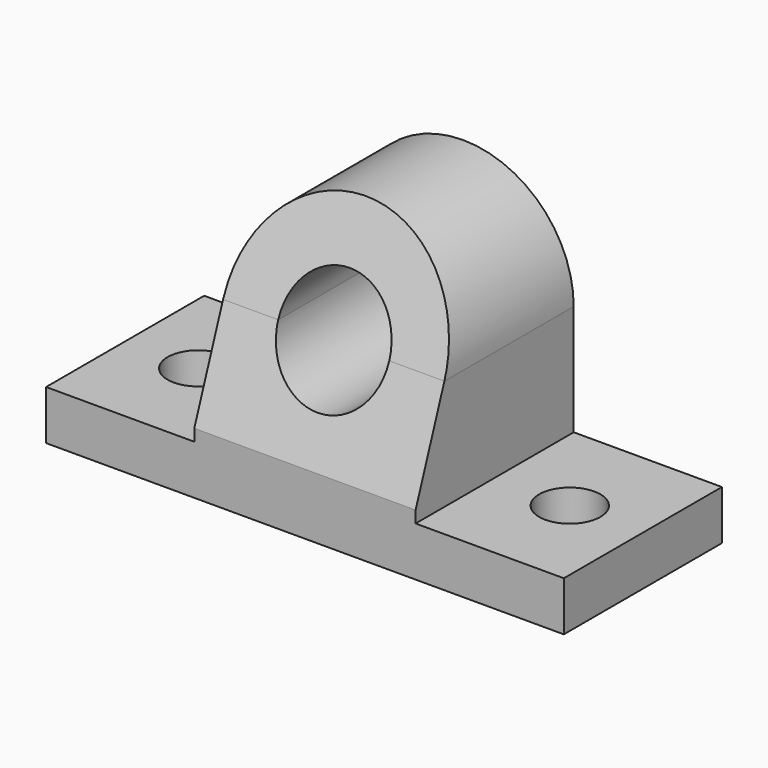
from build123d import *
from build123d import SkipClean  # not in build123d's __all__

# Parameters (mm, degrees)
F1_DEPTH  = 12.7
F2_DEPTH  = 15.748
F3_W      = 56.896
F3_H      = 50.8
F4_DEPTH  = 25.4
F5_DEPTH  = 47.244
F7_DEPTH  = 50.8
F8_DEPTH  = 50.8
F10_DEPTH = 101.6


# Not quite as in the source:
# - a feature names something its author has since deleted; it is built from what else it names


with BuildPart() as f1:
    # F0 (on Top) → F1 (new body)
    with BuildSketch(Plane.XY):
        Polygon((133.096, 50.8), (94.996, 50.8), (94.996, 0), (114.3, 0), (133.096, 0), align=None)
        with BuildLine():
            ThreePointArc((122.174, 25.4), (119.8677587951, 19.8322412049), (114.3, 17.526))
            ThreePointArc((114.3, 17.526), (108.7322412049, 30.9677587951), (122.174, 25.4))
        make_face(mode=Mode.SUBTRACT)
        Polygon((0, 50.8), (0, 0), (18.796, 0), (38.1, 0), (38.1, 50.8), align=None)
        with BuildLine():
            ThreePointArc((26.67, 25.4), (24.3637587951, 19.8322412049), (18.796, 17.526))
            ThreePointArc((18.796, 17.526), (13.2282412049, 30.9677587951), (26.67, 25.4))
        make_face(mode=Mode.SUBTRACT)
        Polygon((94.996, 50.8), (38.1, 50.8), (38.1, 0), (66.548, 0), (94.996, 0), align=None)
    extrude(amount=F1_DEPTH)

    # F0 (on Top) → F2 (join)
    with BuildSketch(Plane.XY):
        Polygon((94.996, 50.8), (38.1, 50.8), (38.1, 0), (66.548, 0), (94.996, 0), align=None)
    extrude(amount=F2_DEPTH)

    # F3 (on face) → F4 (join)
    with BuildSketch(Plane.XY.offset(15.748)):
        with Locations((66.548, 25.4)):
            Rectangle(F3_W, F3_H)
    extrude(amount=F4_DEPTH)

    # F0 (on Top) → F5 (cut)
    with BuildSketch(Plane.XY):
        with BuildLine():
            ThreePointArc((26.67, 25.4), (13.2282412049, 30.9677587951), (18.796, 17.526))
            ThreePointArc((18.796, 17.526), (24.3637587951, 19.8322412049), (26.67, 25.4))
        make_face()
        with BuildLine():
            ThreePointArc((122.174, 25.4), (108.7322412049, 30.9677587951), (114.3, 17.526))
            ThreePointArc((114.3, 17.526), (119.8677587951, 19.8322412049), (122.174, 25.4))
        make_face()
    extrude(amount=-F5_DEPTH, mode=Mode.SUBTRACT)

    # F6 (on face) → F7 (join)
    with BuildSketch(Plane(origin=(0, 50.8, 0), x_dir=(-1, 0, 0), z_dir=(0, 1, 0))):
        with BuildLine():
            Line((-52.2732, 41.148), (-38.1, 41.148))
            ThreePointArc((-38.1, 41.148), (-66.548, 69.596), (-94.996, 41.148))
            Line((-94.996, 41.148), (-80.8228, 41.148))
            ThreePointArc((-80.8228, 41.148), (-66.548, 55.4228), (-52.2732, 41.148))
        make_face()
        with BuildLine():
            ThreePointArc((-94.996, 41.148), (-66.548, 12.7), (-38.1, 41.148))
            Line((-38.1, 41.148), (-52.2732, 41.148))
            ThreePointArc((-52.2732, 41.148), (-66.548, 26.8732), (-80.8228, 41.148))
            Line((-80.8228, 41.148), (-94.996, 41.148))
        make_face()
    extrude(amount=-F7_DEPTH)

    # F6 (on face) → F8 (cut)
    with BuildSketch(Plane(origin=(0, 50.8, 0), x_dir=(-1, 0, 0), z_dir=(0, 1, 0))):
        with BuildLine():
            ThreePointArc((-80.8228, 41.148), (-66.548, 26.8732), (-52.2732, 41.148))
            Line((-52.2732, 41.148), (-80.8228, 41.148))
        make_face()
    with SkipClean():  # cleaning this boolean's faces spoils the solid; the shape is the same uncleaned
        extrude(amount=-F8_DEPTH, mode=Mode.SUBTRACT)

    # F9 (on face) → F10 (cut)
    with BuildSketch(Plane.YZ.offset(94.996)):
        Polygon((0, 68.7535953361), (0, 41.148), (9.2448439504, 41.148), (25.583601225, 86.0383666739), (0, 86.0383666739), align=None)
        Polygon((0, 41.148), (0, 15.748), (9.2448439504, 41.148), align=None)
    with SkipClean():  # cleaning this boolean's faces spoils the solid; the shape is the same uncleaned
        extrude(amount=-F10_DEPTH, mode=Mode.SUBTRACT)


solid = f1.part
